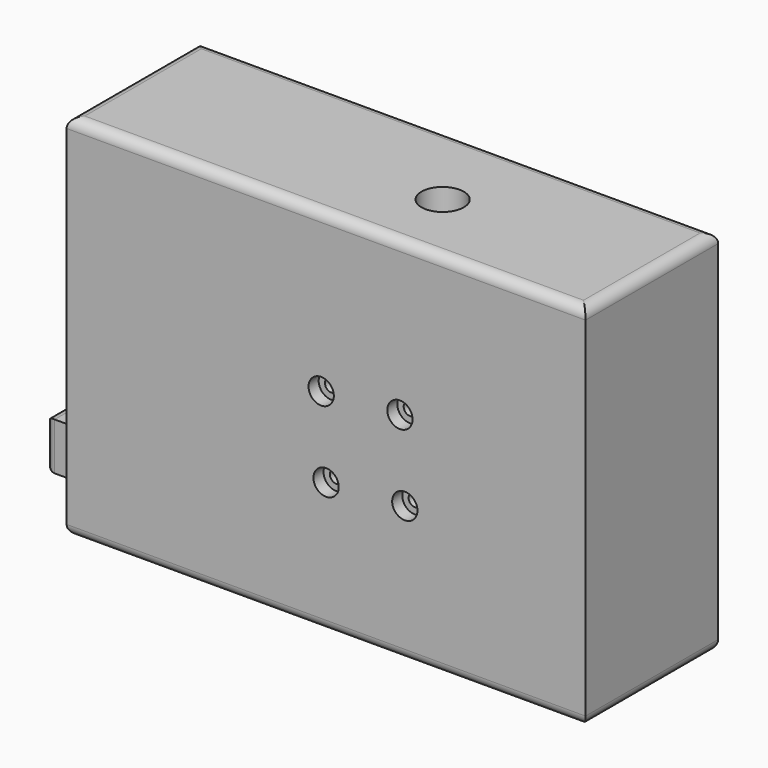
from build123d import *

# Parameters (mm, degrees)
F0_W            = 260.7417907566
F0_H            = 185.2982528508
F1_DEPTH        = 83.312
F2_R            = 5.08
F3_R            = 10.6560791483
F4_DEPTH        = 185.2982528508
F6_DEPTH        = 25.4
F7_R            = 5.08
F9_D            = 6.35
F9_CBORE_D      = 12.7
F9_CBORE_DEPTH  = 6.35
F9_COPIES_COUNT = 4


# Not quite as in the source:
# - a pattern or mirror of a feature is missing from the dataset's text; its kind, count and spacing are read off the source's solid


with BuildPart() as f1:
    # F0 (on Front) → F1 (new body)
    with BuildSketch(Plane.XZ):
        with Locations((-18.5430413112, 5.6122671813)):
            Rectangle(F0_W, F0_H)
    extrude(amount=F1_DEPTH)

    # F2
    f2_edges = [f1.edges().sort_by_distance(p)[0] for p in [
        (-148.913937, -41.656, 98.261394),
        (-18.543041, -83.312, 98.261394),
        (111.827854, -41.656, 98.261394),
        (-18.543041, 0, 98.261394),
    ]]
    fillet(f2_edges, radius=F2_R)

    # F3 (on face) → F4 (cut, through all)
    with BuildSketch(Plane.XY.offset(98.2613936067)):
        with Locations((10.0774681196, -45.8871424198)):
            Circle(F3_R)
    extrude(amount=-F4_DEPTH, mode=Mode.SUBTRACT)

    # F5 (on face) → F6 (join)
    with BuildSketch(Plane(origin=(-148.9139366895, 0, 0), x_dir=(0, -1, 0), z_dir=(-1, 0, 0))):
        with BuildLine():
            ThreePointArc((39.8253589774, -49.4220387191), (36.2562578791, -48.3240875907), (33.9213925534, -45.4099181994))
            ThreePointArc((33.9213925534, -45.4099181994), (16.0837066862, -41.7163656596), (19.777259226, -59.5540515267))
            ThreePointArc((19.777259226, -59.5540515267), (22.6914286173, -61.8889168524), (23.7893797457, -65.4580179507))
            Line((23.7893797457, -65.4580179507), (23.7893797457, -73.2655222528))
            Line((23.7893797457, -73.2655222528), (65.4315222055, -73.2655222528))
            Line((65.4315222055, -73.2655222528), (65.4315222055, -49.4220387191))
            Line((65.4315222055, -49.4220387191), (39.8253589774, -49.4220387191))
        make_face()
    extrude(amount=F6_DEPTH)

    # F7
    f7_edges = [f1.edges().sort_by_distance(p)[0] for p in [
        (-174.313937, -65.431522, -61.34378),
        (-174.313937, -52.628441, -49.422039),
        (-174.313937, -36.256258, -48.324088),
        (-174.313937, -16.083707, -41.716366),
        (-174.313937, -22.691429, -61.888917),
        (-174.313937, -23.78938, -69.36177),
        (-174.313937, -44.610451, -73.265522),
        (-148.913937, -41.656, -87.036859),
        (-18.543041, 0, -87.036859),
        (-18.543041, -83.312, -87.036859),
        (111.827854, -41.656, -87.036859),
        (-0.578611, -45.887142, -87.036859),
    ]]
    fillet(f7_edges, radius=F7_R)

    # F9 (through all)
    with Locations(Plane.XZ.offset(83.312)):
        with Locations((-18.5430413112, -21.0058055818)):
            f9 = CounterBoreHole(F9_D / 2, F9_CBORE_D / 2, F9_CBORE_DEPTH)

    # F9_copies: F9 ×4 about axis
    f9_copies_axis = Axis((0, 0, 0), (0, 1, 0))
    for i in range(1, F9_COPIES_COUNT):
        add(f9.rotate(f9_copies_axis, i * 360 / F9_COPIES_COUNT), mode=Mode.SUBTRACT)


solid = f1.part
